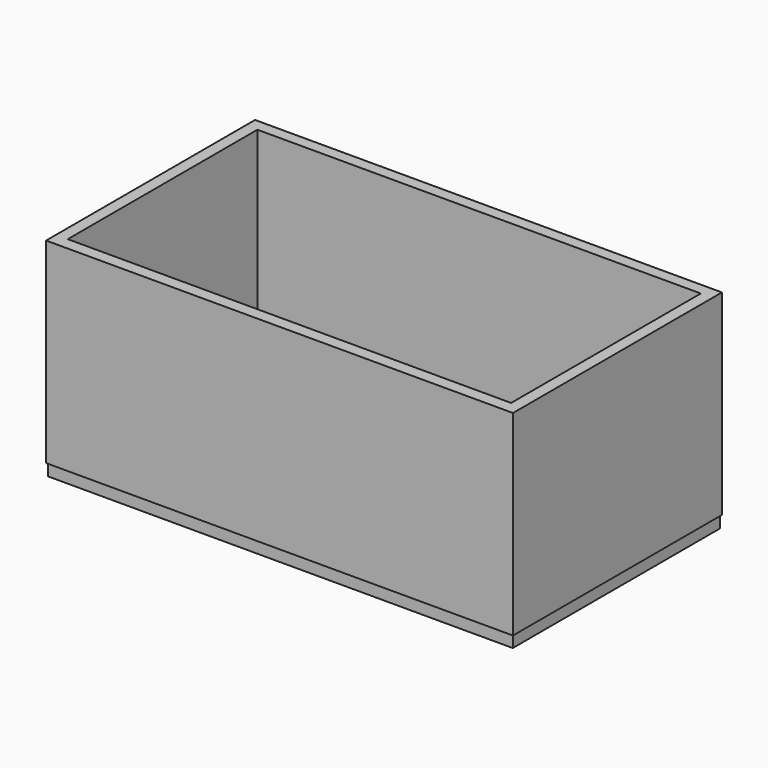
from build123d import *

# Parameters (mm, degrees)
F1_DEPTH = 400
F0_W     = 679
F0_H     = 300
F2_DEPTH = 18
F4_W     = 679
F4_H     = 300
F5_DEPTH = 19
F8_DEPTH = 397


with BuildPart() as f1:
    # F0 (on Front) → F1 (new body)
    with BuildSketch(Plane.XZ):
        Polygon((-356, -150), (-339.5, -150), (-339.5, 150), (-357.5, 150), (-357.5, -150), align=None)
    extrude(amount=F1_DEPTH)



with BuildPart() as f1b:
    # F0 (on Front) → F1, piece 2 (new body)
    with BuildSketch(Plane.XZ):
        Polygon((339.5, 150), (339.5, -150), (356, -150), (357.5, -150), (357.5, 150), align=None)
    extrude(amount=F1_DEPTH)


with BuildPart() as f1_1:
    add(f1.part)

    add(f1b.part)  # F2 merges F1b
    # F0 (on Front) → F2 (join)
    with BuildSketch(Plane.XZ):
        Rectangle(F0_W, F0_H)
    extrude(amount=F2_DEPTH)

    # F4 (on offset) → F5 (join)
    with BuildSketch(Plane.XZ.offset(400)):
        Rectangle(F4_W, F4_H)
    extrude(amount=-F5_DEPTH)


with BuildPart() as f8:
    # F7 (on offset) → F8 (new body)
    with BuildSketch(Plane.XZ.offset(398.5)):
        Polygon((339.5, -150), (-339.5, -150), (-356, -150), (-356, -168), (356, -168), (356, -150), align=None)
    extrude(amount=-F8_DEPTH)


solid = Compound([f1_1.part, f8.part])
